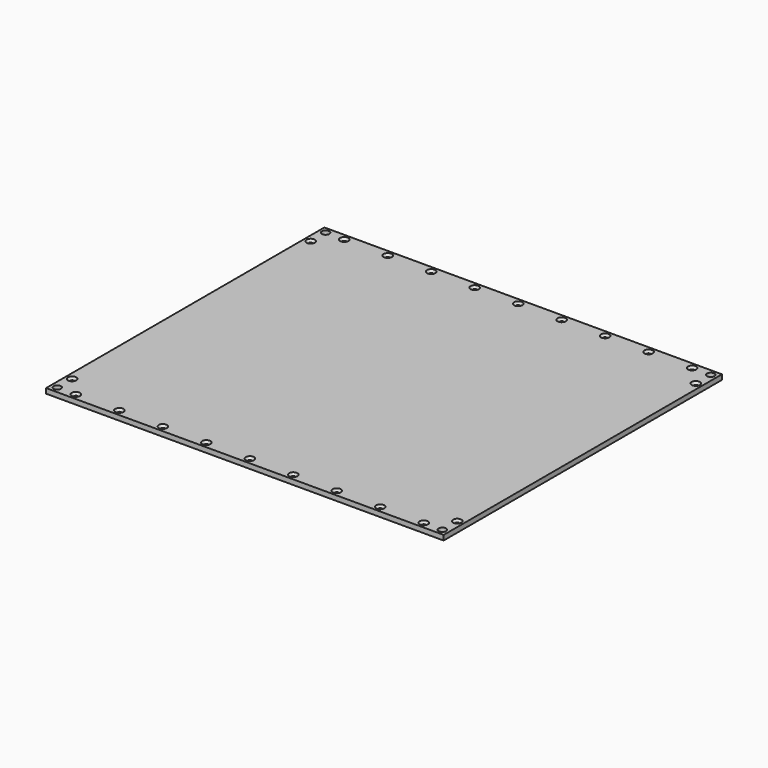
from build123d import *

# Parameters (mm, degrees)
F0_W           = 320
F0_H           = 280
F0_R           = 3
F1_DEPTH       = 4
F2_D           = 3.2
F2_CSINK_D     = 6.72
F2_CSINK_ANGLE = 90


# Not quite as in the source:
# - a feature names something its author has since deleted; it is built from what else it names


with BuildPart() as f1:
    # F0 (on Top) → F1 (new body)
    with BuildSketch(Plane.XY):
        Rectangle(F0_W, F0_H)
        with Locations((-155, -135)):
            Circle(F0_R, mode=Mode.SUBTRACT)
        with Locations((155, -135)):
            Circle(F0_R, mode=Mode.SUBTRACT)
        with Locations((-155, 135)):
            Circle(F0_R, mode=Mode.SUBTRACT)
        with Locations((155, 135)):
            Circle(F0_R, mode=Mode.SUBTRACT)
    extrude(amount=-F1_DEPTH)

    # F2 (through all)
    with Locations(Plane.XY):
        with Locations((0, -135), (0, 135), (-105, 135), (-70, 135), (-35, 135), (35, 135), (70, 135), (105, 135), (-105, -135), (-70, -135), (-35, -135), (35, -135), (70, -135), (105, -135), (140, 135), (140, -135), (-140, 135), (-140, -135), (155, -120), (155, 120), (-155, 120), (-155, -120)):
            CounterSinkHole(F2_D / 2, F2_CSINK_D / 2, counter_sink_angle=F2_CSINK_ANGLE)


solid = f1.part
